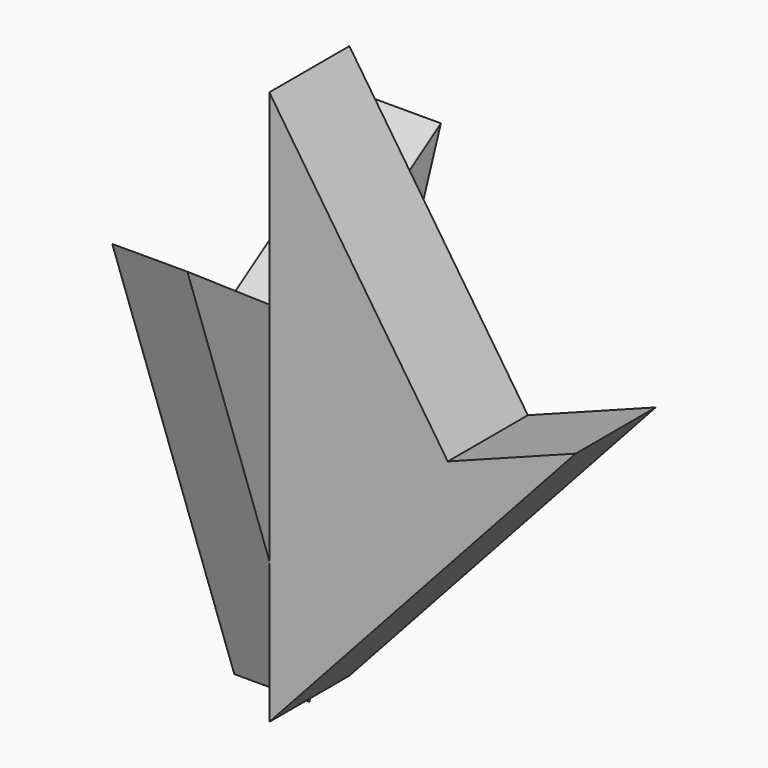
from build123d import *

# Parameters (mm, degrees)
F2_DEPTH      = 15
F3_DEPTH      = 10
F3_DEPTH_BACK = 10


# Not quite as in the source:
# - a feature names something its author has since deleted; it is built from what else it names


with BuildPart() as f2:
    # F1 (on Right) → F2 (new body)
    with BuildSketch(Plane.YZ):
        Polygon((32.8475944698, 30.4612312466), (0, 9.1243321076), (-30.4703023285, 30.1044266671), (0, -57.9494014382), align=None)
    extrude(amount=-F2_DEPTH)

    # F0 (on Front) → F3 (join, two sides)
    with BuildSketch(Plane.XZ) as f3_sk:
        Polygon((35.6550849974, 0), (0, 53.336199373), (0, -57.4131049216), (61.2032115459, 9.6858292818), align=None)
    extrude(amount=-F3_DEPTH)
    extrude(f3_sk.sketch, amount=F3_DEPTH_BACK)


solid = f2.part
